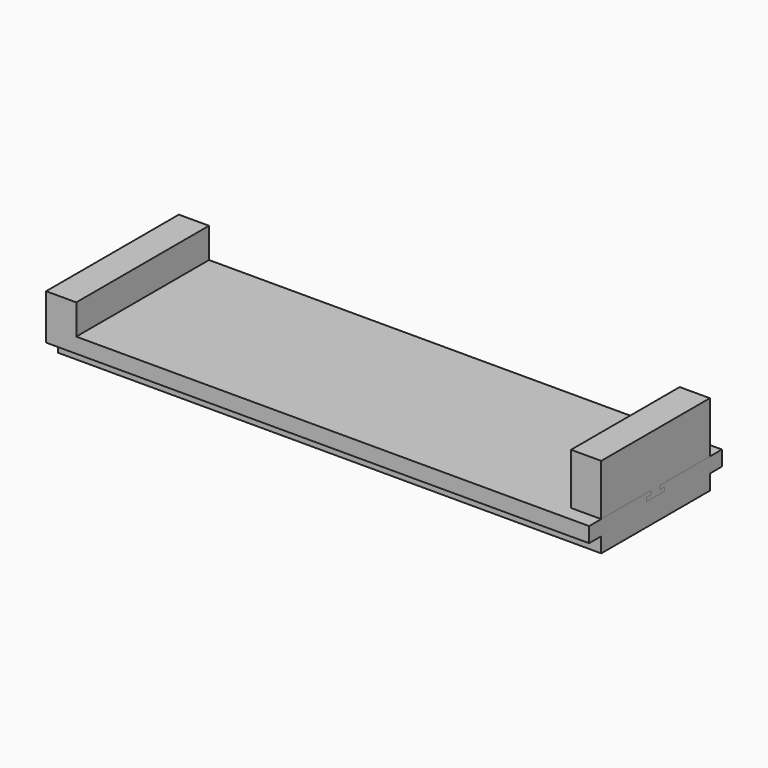
from build123d import *

# Parameters (mm, degrees)
F0_W          = 1
F0_H          = 1
F1_DEPTH      = 32
F1_DEPTH_BACK = 4
F2_W          = 2
F2_H          = 9
F3_DEPTH      = 3.4
F5_DEPTH      = 1
F6_DEPTH      = 1
F7_W          = 2
F7_H          = 11
F8_DEPTH      = 2


with BuildPart() as f1:
    # F0 (on Right) → F1 (new body, two sides)
    with BuildSketch(Plane.YZ) as f1_sk:
        Polygon((4.5, 1), (4.5, 2), (-4.5, 2), (-4.5, 1), (-4.5, 0), (4.5, 0), align=None)
        with Locations((5, 1.5)):
            Rectangle(F0_W, F0_H)
        with Locations((-5, 1.5)):
            Rectangle(F0_W, F0_H)
    extrude(amount=F1_DEPTH)
    extrude(f1_sk.sketch, amount=-F1_DEPTH_BACK)

    # F4 (on face) → F5 (cut)
    with BuildSketch(Plane.YZ.offset(32)):
        Polygon((0.375, 2), (-0.375, 2), (-0.375, 1.75), (-0.75, 1.75), (-0.75, 1.5), (0.75, 1.5), (0.75, 1.75), (0.375, 1.75), align=None)
    extrude(amount=-F5_DEPTH, mode=Mode.SUBTRACT)

    # F7 (on face) → F8 (join)
    with BuildSketch(Plane.XY.offset(2)):
        with Locations((-3, 0)):
            Rectangle(F7_W, F7_H)
    extrude(amount=F8_DEPTH)


with BuildPart() as f3:
    # F2 (on face) → F3 (new body)
    with BuildSketch(Plane.XY.offset(2)):
        with Locations((31, 0)):
            Rectangle(F2_W, F2_H)
    extrude(amount=F3_DEPTH)

    # F4 (on face) → F6 (join)
    with BuildSketch(Plane.YZ.offset(32)):
        Polygon((0.375, 2), (-0.375, 2), (-0.375, 1.75), (-0.75, 1.75), (-0.75, 1.5), (0.75, 1.5), (0.75, 1.75), (0.375, 1.75), align=None)
    extrude(amount=-F6_DEPTH)


solid = Compound([f1.part, f3.part])
